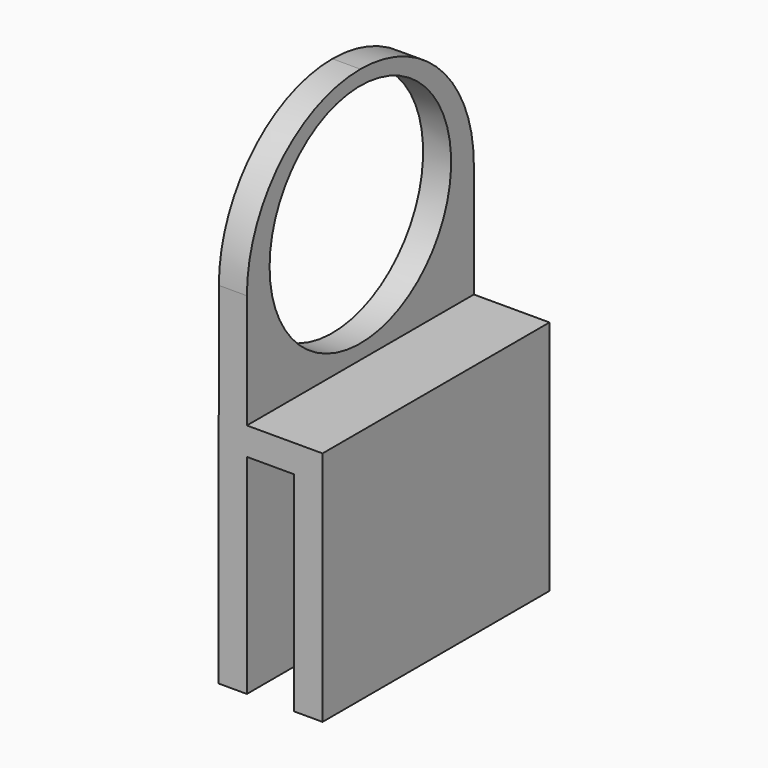
from build123d import *

# Parameters (mm, degrees)
F1_DEPTH = 30
F2_R     = 12
F3_DEPTH = 25
F4_R     = 14.99999
F5_DEPTH = 7.3296


# Not quite as in the source:
# - a fillet or chamfer is up to 0.001 mm smaller than in the source, because OpenCascade refuses the exact size


with BuildPart() as f1:
    # F0 (on Front) → F1 (new body)
    with BuildSketch(Plane.XZ):
        Polygon((-18.8925201073, 27.8060024955), (-18.9275150057, 27.8060024955), (-18.9275150057, 2.8060024955), (-15.9275150057, 2.8060024955), (-15.9275150057, 24.8831361532), (-10.9275150057, 24.8831361532), (-10.9275150057, 2.8060024955), (-7.9275150057, 2.8060024955), (-7.9275150057, 27.8060024955), (-10.9275150057, 27.8060024955), (-15.9275150057, 27.8060024955), (-15.9275150057, 54.8831361532), (-18.8925201073, 54.8831361532), align=None)
    extrude(amount=F1_DEPTH)

    # F2 (on face) → F3 (cut)
    with BuildSketch(Plane(origin=(-18.8925201073, 0, 0), x_dir=(0, -1, 0), z_dir=(-1, 0, 0))):
        with Locations((15, 41.3446361532)):
            Circle(F2_R)
    extrude(amount=-F3_DEPTH, mode=Mode.SUBTRACT)

    # F4 (radius 15 in the source; OpenCascade refuses exactly that, so slightly less here)
    f4_edges = [f1.edges().sort_by_distance(p)[0] for p in [
        (-17.410018, 0, 54.883136),
        (-17.410018, -30, 54.883136),
    ]]
    fillet(f4_edges, radius=F4_R)

    # F2 (on face) → F5 (cut)
    with BuildSketch(Plane(origin=(-18.8925201073, 0, 0), x_dir=(0, -1, 0), z_dir=(-1, 0, 0))):
        with Locations((15, 41.3446361532)):
            Circle(F2_R)
    extrude(amount=-F5_DEPTH, mode=Mode.SUBTRACT)


solid = f1.part
